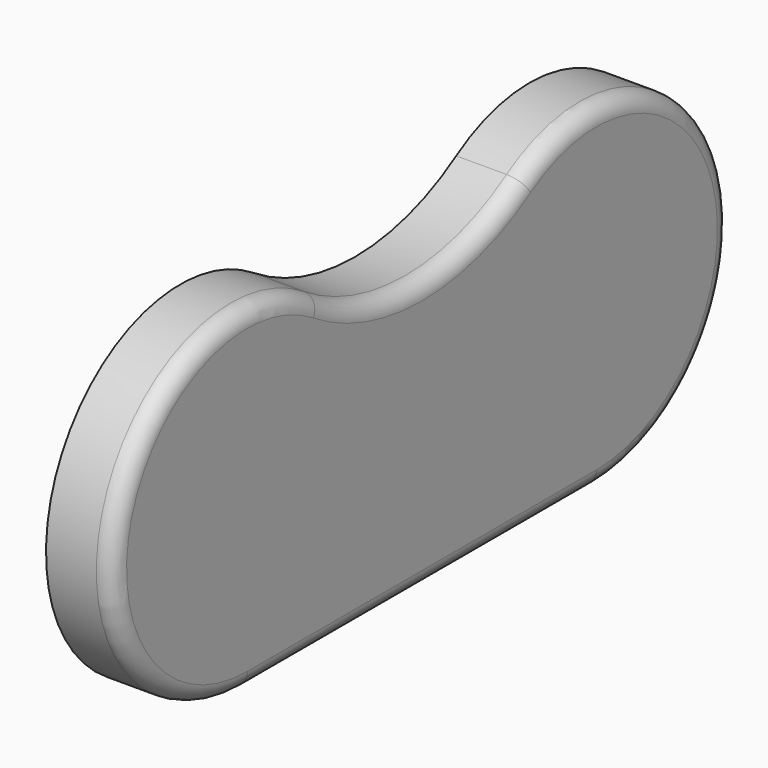
from build123d import *

# Parameters (mm, degrees)
F0_R           = 5.55625
F1_DEPTH       = 47.625
F0_R_2         = 6.5484375
F2_DEPTH       = 19.05
F4_DEPTH       = 28.575
F5_W           = 8.73125
F5_H           = 8.73125
F6_DEPTH       = 47.626
F7_R           = 4.365625
F8_DEPTH       = 9.525
F8_DEPTH_BACK  = 9.525
F10_DEPTH      = 9.525
F12_D          = 2.7051
F12_DEPTH      = 15.875
F12_TIP        = 0.8126940303
F14_DEPTH      = 3.175
F15_W          = 60.325
F15_H          = 50.8
F16_DEPTH      = 25.4
F16_DEPTH_BACK = 8.73225
F18_DEPTH      = 1.5875
F19_R          = 0.79375
F21_DEPTH      = 1.5875
F22_R          = 0.79375


# Not quite as in the source:
# - a pattern or mirror of a feature is missing from the dataset's text; its kind, count and spacing are read off the source's solid
# - a feature names something its author has since deleted; it is built from what else it names


with BuildPart() as f1:
    # F0 (on Right) → F1 (new body)
    with BuildSketch(Plane.YZ):
        with BuildLine():
            ThreePointArc((18.25625, -15.875), (16.6494169978, -11.0868310793), (12.4794785699, -8.2372543707))
            ThreePointArc((12.4794785699, -8.2372543707), (2.4565457231, -14.7842891497), (10.31875, -23.8125))
            ThreePointArc((10.31875, -23.8125), (15.9314100757, -21.4876600757), (18.25625, -15.875))
        make_face()
        with Locations((10.31875, -15.875)):
            Circle(F0_R, mode=Mode.SUBTRACT)
    extrude(amount=F1_DEPTH)



with BuildPart() as f1b:
    # F0 (on Right) → F1, piece 2 (new body)
    with BuildSketch(Plane.YZ):
        with BuildLine():
            ThreePointArc((-2.38125, -15.875), (-5.5305810793, -9.5443330022), (-12.4794785699, -8.2372543707))
            ThreePointArc((-12.4794785699, -8.2372543707), (-18.1809542769, -16.9657108503), (-10.31875, -23.8125))
            ThreePointArc((-10.31875, -23.8125), (-4.7060899243, -21.4876600757), (-2.38125, -15.875))
        make_face()
        with Locations((-10.31875, -15.875)):
            Circle(F0_R, mode=Mode.SUBTRACT)
    extrude(amount=F1_DEPTH)


with BuildPart() as f1_1:
    add(f1.part)

    add(f1b.part)  # F2 merges F1b
    # F0 (on Right) → F2 (join)
    with BuildSketch(Plane.YZ):
        with BuildLine():
            ThreePointArc((8.5506596809, -1.7666198185), (8.6859850881, -0.8879130653), (8.73125, 0))
            ThreePointArc((8.73125, 0), (-0.8879130653, 8.6859850881), (-8.5506596809, -1.7666198185))
            ThreePointArc((-8.5506596809, -1.7666198185), (0, -8.73125), (8.5506596809, -1.7666198185))
        make_face()
        Circle(F0_R_2, mode=Mode.SUBTRACT)
        with BuildLine():
            ThreePointArc((8.5506596809, -1.7666198185), (0, -8.73125), (-8.5506596809, -1.7666198185))
            ThreePointArc((-8.5506596809, -1.7666198185), (-9.2426468573, -5.7745223181), (-12.4794785699, -8.2372543707))
            ThreePointArc((-12.4794785699, -8.2372543707), (-5.5305810793, -9.5443330022), (-2.38125, -15.875))
            ThreePointArc((-2.38125, -15.875), (-4.7060899243, -21.4876600757), (-10.31875, -23.8125))
            Line((-10.31875, -23.8125), (10.31875, -23.8125))
            ThreePointArc((10.31875, -23.8125), (2.4565457231, -14.7842891497), (12.4794785699, -8.2372543707))
            ThreePointArc((12.4794785699, -8.2372543707), (9.2426468573, -5.7745223181), (8.5506596809, -1.7666198185))
        make_face()
    extrude(amount=F2_DEPTH)

    # F3 (on face) → F4 (join, through all)
    with BuildSketch(Plane.YZ.offset(47.625)):
        with BuildLine():
            ThreePointArc((5.9929049671, -9.2198537956), (0, -10.9963909515), (-5.9929049671, -9.2198537956))
            ThreePointArc((-5.9929049671, -9.2198537956), (-3.3423504559, -12.0890053287), (-2.38125, -15.875))
            ThreePointArc((-2.38125, -15.875), (-4.7060899243, -21.4876600757), (-10.31875, -23.8125))
            Line((-10.31875, -23.8125), (10.31875, -23.8125))
            ThreePointArc((10.31875, -23.8125), (2.7085880685, -18.1309569203), (5.9929049671, -9.2198537956))
        make_face()
    extrude(amount=-F4_DEPTH)

    # F5 (on face) → F6 (cut, through all)
    with BuildSketch(Plane(origin=(0, 0, 0), x_dir=(0, -1, 0), z_dir=(-1, 0, 0))):
        with Locations((0, -16.271875)):
            Rectangle(F5_W, F5_H)
    extrude(amount=-F6_DEPTH, mode=Mode.SUBTRACT)

    # F7 (on Front) → F8 (cut, two sides)
    with BuildSketch(Plane.XZ) as f8_sk:
        with Locations((0, -16.271875)):
            Circle(F7_R)
        with Locations((47.625, -16.271875)):
            Circle(F7_R)
    extrude(amount=-F8_DEPTH, mode=Mode.SUBTRACT)
    extrude(f8_sk.sketch, amount=F8_DEPTH_BACK, mode=Mode.SUBTRACT)

    # F9 (on face) → F10 (cut)
    with BuildSketch(Plane(origin=(0, 0, -11.90625), x_dir=(1, 0, 0), z_dir=(0, 0, -1))):
        with BuildLine():
            ThreePointArc((0, -4.3352987234), (2.7498472571, -2.8996680512), (3.8519455094, 0))
            ThreePointArc((3.8519455094, 0), (2.7498472571, 2.8996680512), (0, 4.3352987234))
            Line((0, 4.3352987234), (0, -4.3352987234))
        make_face()
        with BuildLine():
            Line((0, -4.3352987234), (0, 4.3352987234))
            ThreePointArc((0, 4.3352987234), (-4.8793044906, 0), (0, -4.3352987234))
        make_face()
    extrude(amount=-F10_DEPTH, mode=Mode.SUBTRACT)

    # F12
    with Locations(Plane(origin=(0, 0, 0), x_dir=(0, -1, 0), z_dir=(-1, 0, 0))):
        with Locations((7.14375, -7.9375), (-7.14375, -7.9375)):
            Hole(F12_D / 2, depth=F12_DEPTH)
            with Locations((0, 0, -(F12_DEPTH + F12_TIP / 2))):  # 118° drill point
                Cone(0, F12_D / 2, F12_TIP, mode=Mode.SUBTRACT)

    # F13 (on face) → F14 (join)
    with BuildSketch(Plane.YZ.offset(47.625)):
        with BuildLine():
            ThreePointArc((5.9929049671, -9.2198537956), (0, -10.9963909515), (-5.9929049671, -9.2198537956))
            ThreePointArc((-5.9929049671, -9.2198537956), (-17.9289119315, -13.6190430797), (-10.31875, -23.8125))
            Line((-10.31875, -23.8125), (10.31875, -23.8125))
            ThreePointArc((10.31875, -23.8125), (17.9289119315, -13.6190430797), (5.9929049671, -9.2198537956))
        make_face()
        with BuildLine():
            ThreePointArc((-7.4568436751, -20.6375), (-15.8369831688, -15.2261419591), (-6.4301850333, -11.90625))
            Line((-6.4301850333, -11.90625), (-4.365625, -11.90625))
            Line((-4.365625, -11.90625), (4.365625, -11.90625))
            Line((4.365625, -11.90625), (6.4301850333, -11.90625))
            ThreePointArc((6.4301850333, -11.90625), (12.4711991825, -10.7526102668), (15.875, -15.875))
            ThreePointArc((15.875, -15.875), (13.054663654, -20.7109787572), (7.4568436751, -20.6375))
            Line((7.4568436751, -20.6375), (4.365625, -20.6375))
            Line((4.365625, -20.6375), (-4.365625, -20.6375))
            Line((-4.365625, -20.6375), (-7.4568436751, -20.6375))
        make_face(mode=Mode.SUBTRACT)
        with BuildLine():
            Line((-4.365625, -11.90625), (-6.4301850333, -11.90625))
            ThreePointArc((-6.4301850333, -11.90625), (-15.8369831688, -15.2261419591), (-7.4568436751, -20.6375))
            Line((-7.4568436751, -20.6375), (-4.365625, -20.6375))
            Line((-4.365625, -20.6375), (4.365625, -20.6375))
            Line((4.365625, -20.6375), (7.4568436751, -20.6375))
            ThreePointArc((7.4568436751, -20.6375), (13.054663654, -20.7109787572), (15.875, -15.875))
            ThreePointArc((15.875, -15.875), (12.4711991825, -10.7526102668), (6.4301850333, -11.90625))
            Line((6.4301850333, -11.90625), (4.365625, -11.90625))
            Line((4.365625, -11.90625), (-4.365625, -11.90625))
        make_face()
    extrude(amount=F14_DEPTH)

    # F15 (on Top) → F16 (cut, two sides)
    with BuildSketch(Plane.XY) as f16_sk:
        with Locations((17.4625, 0)):
            Rectangle(F15_W, F15_H)
    extrude(amount=-F16_DEPTH, mode=Mode.SUBTRACT)
    extrude(f16_sk.sketch, amount=F16_DEPTH_BACK, mode=Mode.SUBTRACT)

    # F17 (on face) → F18 (join)
    with BuildSketch(Plane.YZ.offset(47.625)):
        with BuildLine():
            ThreePointArc((-7.4568436751, -20.6375), (-5.4827712428, -18.610913654), (-4.7625, -15.875))
            ThreePointArc((-4.7625, -15.875), (-5.1963602668, -13.7225508175), (-6.4301850333, -11.90625))
            ThreePointArc((-6.4301850333, -11.90625), (-15.8369831688, -15.2261419591), (-7.4568436751, -20.6375))
        make_face()
    f18 = extrude(amount=-F18_DEPTH)

    # F18_copies: F18 across plane
    add(f18.mirror(Plane.ZX))

    # F19
    f19_edges = [f1_1.edges().sort_by_distance(p)[0] for p in [
        (46.0375, 13.180656, -11.1125),
        (46.0375, -13.180656, -11.1125),
    ]]
    fillet(f19_edges, radius=F19_R)

    # F20 (on face) → F21 (cut)
    with BuildSketch(Plane(origin=(46.0375, 0, 0), x_dir=(0, -1, 0), z_dir=(-1, 0, 0))):
        with BuildLine():
            Line((6.7689920857, -12.7), (-12.7, -12.7))
            Line((-12.7, -12.7), (-12.7, -19.05))
            Line((-12.7, -19.05), (6.7689920857, -19.05))
            ThreePointArc((6.7689920857, -19.05), (5.55625, -15.875), (6.7689920857, -12.7))
        make_face()
        with BuildLine():
            Line((12.7, -12.7), (6.7689920857, -12.7))
            ThreePointArc((6.7689920857, -12.7), (5.55625, -15.875), (6.7689920857, -19.05))
            Line((6.7689920857, -19.05), (12.7, -19.05))
            Line((12.7, -19.05), (12.7, -12.7))
        make_face()
    extrude(amount=-F21_DEPTH, mode=Mode.SUBTRACT)

    # F22
    f22_edges = [f1_1.edges().sort_by_distance(p)[0] for p in [
        (50.8, 17.928912, -13.619043),
        (50.8, 0, -10.996391),
        (50.8, -17.928912, -13.619043),
        (50.8, 0, -23.8125),
    ]]
    fillet(f22_edges, radius=F22_R)


solid = f1_1.part
